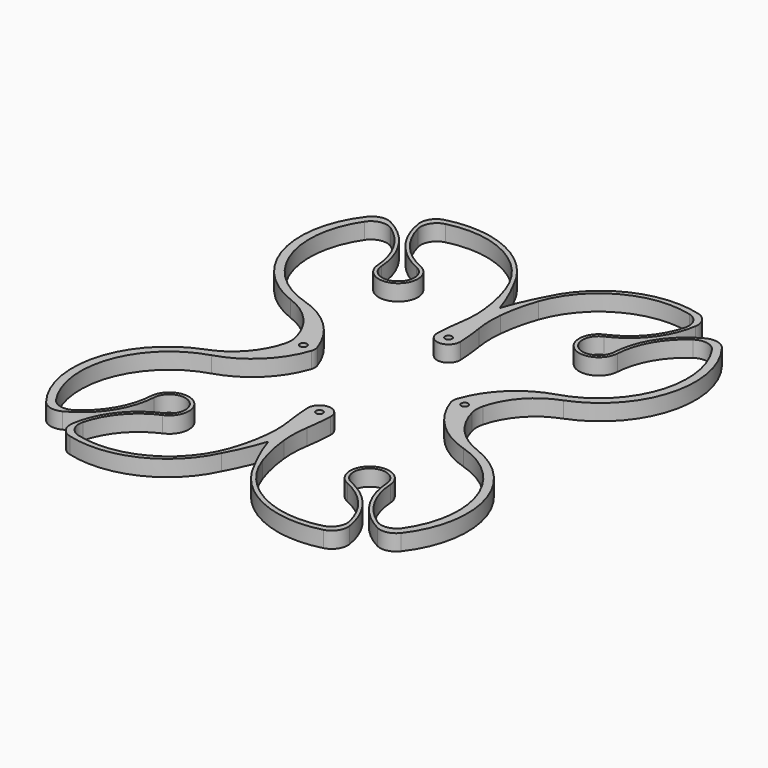
from build123d import *

# Parameters (mm, degrees)
F0_R     = 0.65
F1_DEPTH = 3
F2_R     = 3
F4_R     = 20
F6_R     = 5


with BuildPart() as f1:
    # F0 (on Top) → F1 (new body)
    with BuildSketch(Plane.XY):
        with BuildLine():
            ThreePointArc((3.048863873, 33.9435306954), (-0.6273013424, 24.8132137503), (-2.1481646082, 15.0888190064))
            ThreePointArc((-2.1481646082, 15.0888190064), (0.1920605746, 12.858595616), (2.0980751158, 15.4696603119))
            ThreePointArc((2.0980751158, 15.4696603119), (1.4192789442, 23.8429601845), (3.069932673, 32.0799655424))
            ThreePointArc((3.069932673, 32.0799655424), (12.0601559719, 41.7531852942), (25.2660232668, 41.7340981842))
            ThreePointArc((25.2660232668, 41.7340981842), (22.9072458685, 34.6943477022), (17.1816377079, 29.9678977812))
            ThreePointArc((17.1816377079, 29.9678977812), (16.5476801887, 23.6325364777), (22.284146214, 26.3950828614))
            ThreePointArc((22.284146214, 26.3950828614), (24.7672830036, 33.3919356789), (30.5757351999, 38.016197863))
            ThreePointArc((30.5757351999, 38.016197863), (34.599160335, 22.4278505324), (23.4304919264, 10.8327926069))
            ThreePointArc((23.4304919264, 10.8327926069), (16.96829678, 7.0280687356), (12.9631086037, 0.6881667238))
            ThreePointArc((12.9631086037, 0.6881667238), (14.6512999154, -2.1215344096), (17.15, 0))
            ThreePointArc((17.15, 0), (19.8850375187, 6.1416852415), (25.3777188204, 10.0186918127))
            ThreePointArc((25.3777188204, 10.0186918127), (36.3236498207, 22.8680604315), (31.4714428519, 39.0351803636))
            ThreePointArc((31.4714428519, 39.0351803636), (24.602916766, 34.2580637978), (21.6354084548, 26.4355713753))
            ThreePointArc((21.6354084548, 26.4355713753), (16.9205048724, 24.1649853065), (17.441565847, 29.3721315833))
            ThreePointArc((17.441565847, 29.3721315833), (23.7315501924, 34.7633774873), (25.9233123005, 42.752470948))
            ThreePointArc((25.9233123005, 42.752470948), (12.7075194654, 42.966465136), (3.048863873, 33.9435306954))
        make_face()
        with Locations((15, 0)):
            Circle(F0_R, mode=Mode.SUBTRACT)
        with Locations((0, 15)):
            Circle(F0_R, mode=Mode.SUBTRACT)
    extrude(amount=F1_DEPTH)

    # F2
    f2_edges = [f1.edges().sort_by_distance(p)[0] for p in [
        (30.575735, 38.016198, 1.5),
        (31.471443, 39.03518, 1.5),
        (25.923312, 42.752471, 1.5),
        (25.266023, 41.734098, 1.5),
    ]]
    fillet(f2_edges, radius=F2_R)

    # F3: F1 across plane


with BuildPart() as f1_1:
    add(f1.part)
    add(f1.part.mirror(Plane.YZ))

    # F4
    f4_edges = [f1_1.edges().sort_by_distance(p)[0] for p in [
        (-1.370487, 21.661677, 1.5),
        (1.370487, 21.661677, 1.5),
    ]]
    fillet(f4_edges, radius=F4_R)

    # F5: F1 across plane


with BuildPart() as f1_2:
    add(f1_1.part)
    add(f1_1.part.mirror(Plane.XZ))

    # F6
    f6_edges = [f1_2.edges().sort_by_distance(p)[0] for p in [
        (17.15, 0, 1.5),
        (-17.15, 0, 1.5),
    ]]
    fillet(f6_edges, radius=F6_R)


solid = f1_2.part
